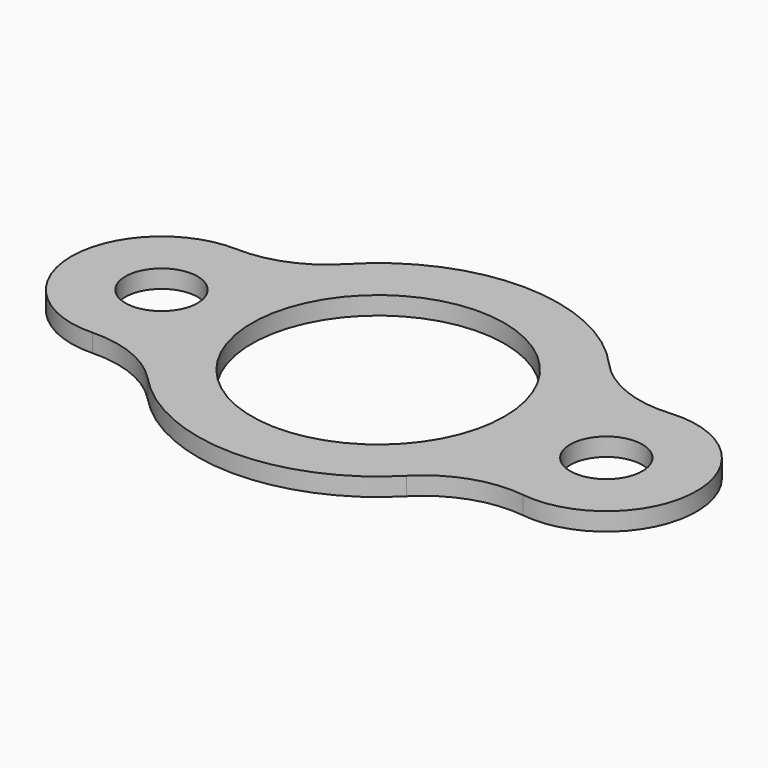
from build123d import *

# Parameters (mm, degrees)
F0_R     = 12.7
F0_R_2   = 44.45
F1_DEPTH = 6.35


# Not quite as in the source:
# - a length typed as a fraction of an inch, garbled in the dataset ("3 / 203.2 mm" for 3/8 in), is restored


with BuildPart() as f1:
    # F0 (on Top) → F1 (new body)
    with BuildSketch(Plane.XY):
        with BuildLine():
            ThreePointArc((-46.13671875, 43.6308741946), (-59.3475236203, 34.5646316236), (-75.1176136364, 31.7315448688))
            ThreePointArc((-75.1176136364, 31.7315448688), (-107.95, 0), (-75.1176136364, -31.7315448688))
            ThreePointArc((-75.1176136364, -31.7315448688), (-59.3475236203, -34.5646316236), (-46.13671875, -43.6308741946))
            ThreePointArc((-46.13671875, -43.6308741946), (-0.5192783502, -63.4978767361), (45.4169792735, -44.3795898321))
            ThreePointArc((45.4169792735, -44.3795898321), (60.1682182179, -35.0158685824), (77.5480268965, -33.2212721562))
            ThreePointArc((77.5480268965, -33.2212721562), (113.3582561105, -2.4068513639), (78.8882291033, 29.8997777276))
            ThreePointArc((78.8882291033, 29.8997777276), (61.6002556172, 32.4304493339), (47.2597573079, 42.4118537581))
            ThreePointArc((47.2597573079, 42.4118537581), (0.8287379603, 63.4945918437), (-46.13671875, 43.6308741946))
        make_face()
        with Locations((81.6154102788, -1.7328791769)):
            Circle(F0_R, mode=Mode.SUBTRACT)
        with Locations((-76.2, 0)):
            Circle(F0_R, mode=Mode.SUBTRACT)
        Circle(F0_R_2, mode=Mode.SUBTRACT)
    extrude(amount=F1_DEPTH)


solid = f1.part
